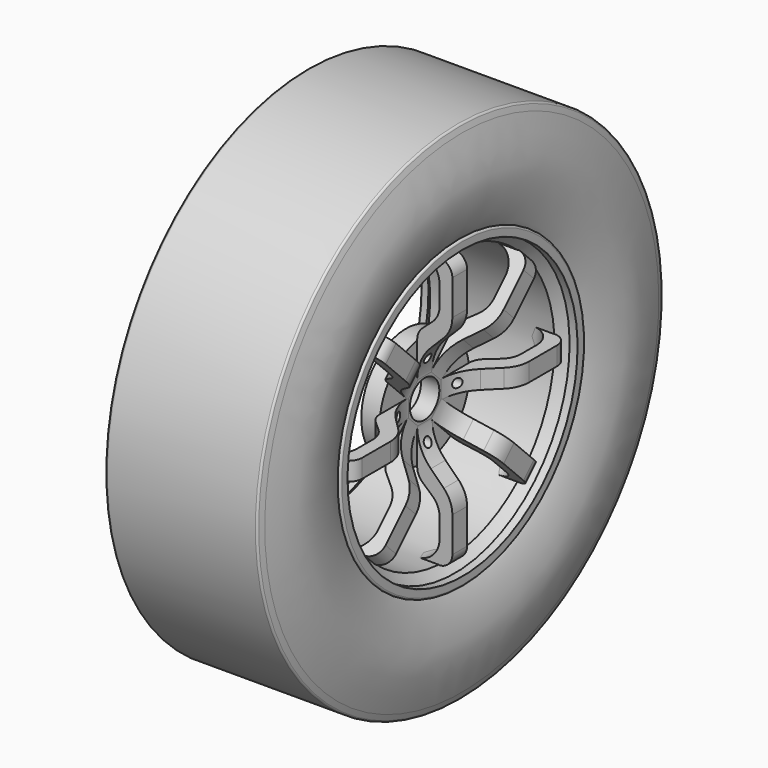
from build123d import *

# Parameters (mm, degrees)
F2_R     = 76
F2_R_2   = 25
F3_DEPTH = 25
F5_DEPTH = 12.5
F6_COUNT = 8
F7_R     = 6
F8_DEPTH = 76.601


with BuildPart() as f1:
    # F0 (on Front) → F1 (revolve)
    with BuildSketch(Plane.XZ):
        with BuildLine():
            Line((-136.6, 205), (-136.6, 197.981321196))
            ThreePointArc((-136.6, 197.981321196), (-135.8363758489, 195.9816654601), (-133.9342512918, 195))
            Line((-133.9342512918, 195), (-125.6710678119, 195))
            Line((-125.6710678119, 195), (-114.3098640222, 183.6387962103))
            Line((-114.3098640222, 183.6387962103), (54.3098640222, 183.6387962103))
            Line((54.3098640222, 183.6387962103), (65.6710678119, 195))
            Line((65.6710678119, 195), (76.4865412602, 195))
            ThreePointArc((76.4865412602, 195), (76.5714999395, 195.4047003657), (76.6, 195.8172389818))
            Line((76.6, 195.8172389818), (76.6, 205))
            ThreePointArc((76.6, 205), (74.1, 207.5), (71.6, 205))
            Line((71.6, 205), (71.6, 202))
            ThreePointArc((71.6, 202), (71.0142135624, 200.5857864376), (69.6, 200))
            Line((69.6, 200), (63.6, 200))
            Line((63.6, 200), (52.2387962103, 188.6387962103))
            Line((52.2387962103, 188.6387962103), (-112.2387962103, 188.6387962103))
            Line((-112.2387962103, 188.6387962103), (-123.6, 200))
            Line((-123.6, 200), (-129.6, 200))
            ThreePointArc((-129.6, 200), (-131.0142135624, 200.5857864376), (-131.6, 202))
            Line((-131.6, 202), (-131.6, 205))
            ThreePointArc((-131.6, 205), (-134.1, 207.5), (-136.6, 205))
        make_face()
    revolve(axis=Axis((-118.9592257142, 0, 0), (-1, 0, 0)))



with BuildPart() as f3:
    # F2 (on Right) → F3 (new body)
    with BuildSketch(Plane.YZ):
        Circle(F2_R)
        Circle(F2_R_2, mode=Mode.SUBTRACT)
    extrude(amount=F3_DEPTH)


with BuildPart() as f1_1:
    add(f1.part)

    add(f3.part)  # F5 merges F3
    # F4 (on Front) → F5 (join, symmetric)
    with BuildSketch(Plane.XZ):
        with BuildLine():
            Line((72.6915134379, 117.7218607421), (72.6915134379, 165.2571467945))
            ThreePointArc((72.6915134379, 165.2571467945), (67.3076529734, 178.2549357458), (54.3098640222, 183.6387962103))
            Line((54.3098640222, 183.6387962103), (23.7416145835, 183.6387962103))
            ThreePointArc((23.7416145835, 183.6387962103), (46.1211403377, 174.3688931234), (55.3910434246, 151.9893673692))
            Line((55.3910434246, 151.9893673692), (55.3910434246, 125.6131570802))
            ThreePointArc((55.3910434246, 125.6131570802), (52.8773311414, 113.8415043444), (45.7746912748, 104.1233221841))
            Line((45.7746912748, 104.1233221841), (32.1275047641, 91.9279629339))
            ThreePointArc((32.1275047641, 91.9279629339), (26.8631281379, 84.7249832003), (25, 76))
            Line((25, 76), (25, 27.6022536848))
            ThreePointArc((25, 27.6022536848), (29.7946982003, 51.7068319755), (43.44884362, 72.1417075136))
            Line((43.44884362, 72.1417075136), (61.1391726256, 89.8320395249))
            ThreePointArc((61.1391726256, 89.8320395249), (69.6891579059, 102.6279985311), (72.6915134379, 117.7218607421))
        make_face()
    extrude(amount=F5_DEPTH, both=True)

    # F6: F1 ×8 about axis
    f6_axis = Axis((25, 0, 0), (1, 0, 0))


with BuildPart() as f1_2:
    add(f1_1.part)
    for i in range(1, F6_COUNT):
        add(f1_1.part.rotate(f6_axis, i * 360 / F6_COUNT))

    # F7 (on Right) → F8 (cut, through all)
    with BuildSketch(Plane.YZ):
        with Locations((0, 50)):
            Circle(F7_R)
        with Locations((-50, 0)):
            Circle(F7_R)
        with Locations((0, -50)):
            Circle(F7_R)
        with Locations((50, 0)):
            Circle(F7_R)
    extrude(amount=F8_DEPTH, mode=Mode.SUBTRACT)


with BuildPart() as f10:
    # F9 (on Front) → F10 (revolve)
    with BuildSketch(Plane.XZ):
        with BuildLine():
            Line((70.2790948941, 343.5), (-130.2790948941, 343.5))
            ThreePointArc((-130.2790948941, 343.5), (-132.0640939314, 342.9111778111), (-133.1483949419, 341.3758522912))
            Line((-133.1483949419, 341.3758522912), (-135.4195076374, 333.9356665075))
            add(Edge.make_bspline(
                [(-131.6, 205), (-132.4705397262, 206.3291423041), (-135.897383717, 211.5612565668), (-154.3296135939, 269.3857359997), (-141.962956636, 311.599505139), (-135.4195076374, 333.9356665075)],
                knots=[0, 0, 0, 0, 0.1381957446, 0.5440018906, 1, 1, 1, 1], degree=3))
            Line((-131.6, 205), (-131.6, 202))
            ThreePointArc((-131.6, 202), (-131.0142135624, 200.5857864376), (-129.6, 200))
            Line((-129.6, 200), (-124.4232303224, 200))
            Line((-124.4232303224, 200), (-124.4232303224, 203.0903667212))
            add(Edge.make_bspline(
                [(-125.813215971, 332.5309753418), (-133.3669424057, 319.600880146), (-143.3729065345, 292.2466144583), (-142.8193701315, 246.9543236386), (-131.3194327453, 208.8816756073), (-128.8000974026, 206.1503215063), (-124.4946131112, 203.8636161095), (-124.4232303224, 203.0903667212)],
                knots=[0, 0, 0, 0, 0.2776874674, 0.5708755502, 0.8259923866, 0.9087323485, 1, 1, 1, 1], degree=3))
            Line((-125.813215971, 332.5309753418), (-30, 332.5309753418))
            Line((-30, 332.5309753418), (65.813215971, 332.5309753418))
            add(Edge.make_bspline(
                [(65.813215971, 332.5309753418), (73.3669424057, 319.600880146), (83.3729065345, 292.2466144583), (82.8193701315, 246.9543236386), (71.3194327453, 208.8816756073), (68.8000974026, 206.1503215063), (64.4946131112, 203.8636161095), (64.4232303224, 203.0903667212)],
                knots=[0, 0, 0, 0, 0.2776874674, 0.5708755502, 0.8259923866, 0.9087323485, 1, 1, 1, 1], degree=3))
            Line((64.4232303224, 203.0903667212), (64.4232303224, 200))
            Line((64.4232303224, 200), (69.6, 200))
            ThreePointArc((69.6, 200), (71.0142135624, 200.5857864376), (71.6, 202))
            Line((71.6, 202), (71.6, 205))
            add(Edge.make_bspline(
                [(71.6, 205), (72.4705397262, 206.3291423041), (75.897383717, 211.5612565668), (94.3296135939, 269.3857359997), (81.962956636, 311.599505139), (75.4195076374, 333.9356665075)],
                knots=[0, 0, 0, 0, 0.1381957446, 0.5440018906, 1, 1, 1, 1], degree=3))
            Line((75.4195076374, 333.9356665075), (73.1483949419, 341.3758522912))
            ThreePointArc((73.1483949419, 341.3758522912), (72.0640939314, 342.9111778111), (70.2790948941, 343.5))
        make_face()
    revolve(axis=Axis((-138.3375376463, 0, 0), (-1, 0, 0)))


solid = Compound([f1_2.part, f10.part])
